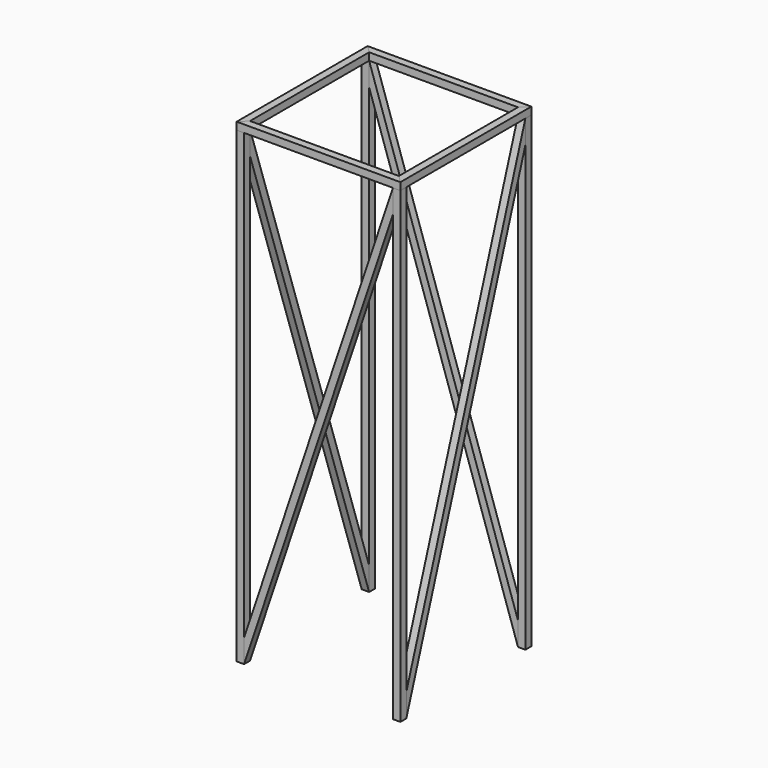
from build123d import *

# Parameters (mm, degrees)
F1_DEPTH = 3.175
F2_DEPTH = 3.175
F3_DEPTH = 3.175
F6_SIZE  = 3.17499
F7_ANGLE = 90
F8_ANGLE = 180


# Not quite as in the source:
# - a fillet or chamfer is up to 0.001 mm smaller than in the source, because OpenCascade refuses the exact size


with BuildPart() as f1:
    # F0 (on Front) → F1 (new body)
    with BuildSketch(Plane.XZ):
        Polygon((3.175, 200), (0, 200), (0, 0), (3.175, 0), (3.175, 190.0045005843), align=None)
    extrude(amount=F1_DEPTH)


with BuildPart() as f2:
    # F0 (on Front) → F2 (new body)
    with BuildSketch(Plane.XZ):
        Polygon((0, 203.175), (0, 200), (3.175, 200), (70, 200), (70, 203.175), align=None)
    extrude(amount=F2_DEPTH)

    # F6 (size 3.175 in the source; OpenCascade refuses exactly that, so slightly less here)
    f6_edges = [f2.edges().sort_by_distance(p)[0] for p in [
        (0, -3.175, 201.5875),
        (70, -3.175, 201.5875),
    ]]
    chamfer(f6_edges, length=F6_SIZE)


with BuildPart() as f3:
    # F0 (on Front) → F3 (new body)
    with BuildSketch(Plane.XZ):
        Polygon((66.825, 9.9954994157), (3.175, 200), (3.175, 190.0045005843), (66.825, 0), align=None)
    extrude(amount=F3_DEPTH)


with BuildPart() as f7_1:
    # F7: copy of F1
    add(f1.part.rotate(Axis((35, -35, 100), (0, 0, -1)), F7_ANGLE))


with BuildPart() as f7_2:
    # F7: copy of F2
    add(f2.part.rotate(Axis((35, -35, 100), (0, 0, -1)), F7_ANGLE))


with BuildPart() as f7_3:
    # F7: copy of F3
    add(f3.part.rotate(Axis((35, -35, 100), (0, 0, -1)), F7_ANGLE))


with BuildPart() as f8_1:
    # F8: copy of F1
    add(f1.part.rotate(Axis((35, -35, 100), (0, 0, -1)), F8_ANGLE))


with BuildPart() as f8_2:
    # F8: copy of F2
    add(f2.part.rotate(Axis((35, -35, 100), (0, 0, -1)), F8_ANGLE))


with BuildPart() as f8_3:
    # F8: copy of F7_1
    add(f7_1.part.rotate(Axis((35, -35, 100), (0, 0, -1)), F8_ANGLE))


with BuildPart() as f8_4:
    # F8: copy of F7_2
    add(f7_2.part.rotate(Axis((35, -35, 100), (0, 0, -1)), F8_ANGLE))


with BuildPart() as f8_5:
    # F8: copy of F3
    add(f3.part.rotate(Axis((35, -35, 100), (0, 0, -1)), F8_ANGLE))


with BuildPart() as f8_6:
    # F8: copy of F7_3
    add(f7_3.part.rotate(Axis((35, -35, 100), (0, 0, -1)), F8_ANGLE))


solid = Compound([f1.part, f2.part, f3.part, f7_1.part, f7_2.part, f7_3.part, f8_1.part, f8_2.part, f8_3.part, f8_4.part, f8_5.part, f8_6.part])
